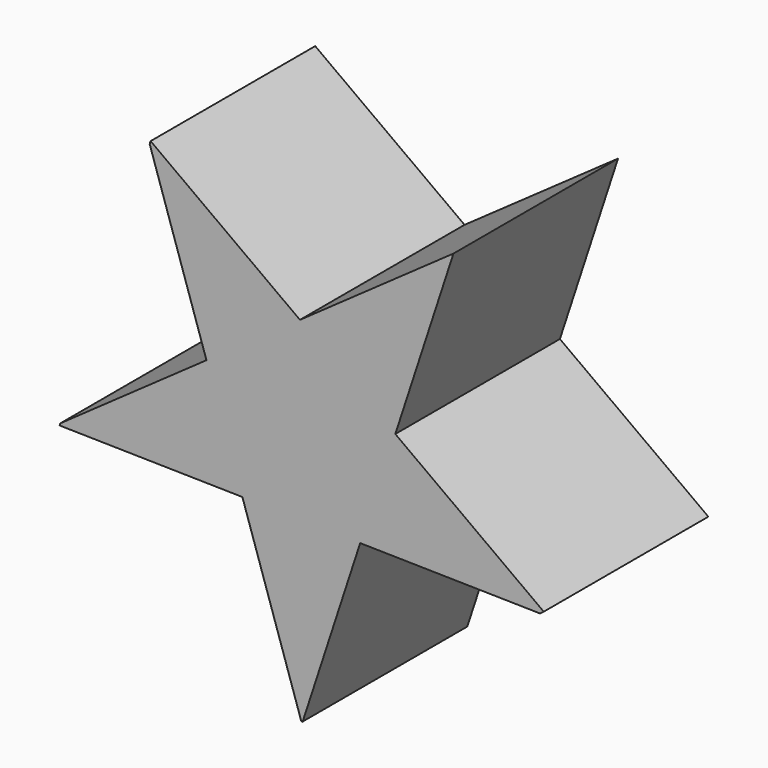
from build123d import *

# Parameters (mm, degrees)
F2_DEPTH = 38.1


with BuildPart() as f2:
    # F1 (on face) → F2 (new body)
    with BuildSketch(Plane.XZ):
        Polygon((0.1359417947, -47.3937628545), (10.7827526257, -14.8319200301), (-11.0337428161, -14.4123720925), (-0.1378061081, -47.3924083515), (0, -47.4925303496), align=None)
        Polygon((44.7767423867, -14.9603227402), (17.2892784216, 5.0674163686), (10.7827526257, -14.8319200301), (44.0723355844, -15.472104239), align=None)
        Polygon((-17.6862078163, 5.7234402568), (-0.3723328356, 17.935905908), (-28.025253062, 38.0841986931), (-28.1999326712, 37.5465901356), align=None)
        Polygon((-11.0337428161, -14.4123720925), (-17.6862078163, 5.7234402568), (-44.7402710109, -13.3593368718), (-44.8709923662, -13.7616558351), align=None)
        Polygon((17.2892784216, 5.0674163686), (28.0526187271, 37.9856489599), (-0.3723328356, 17.935905908), align=None)
        Polygon((10.7827526257, -14.8319200301), (17.2892784216, 5.0674163686), (-0.3723328356, 17.935905908), (-17.6862078163, 5.7234402568), (-11.0337428161, -14.4123720925), align=None)
    extrude(amount=F2_DEPTH)


solid = f2.part
